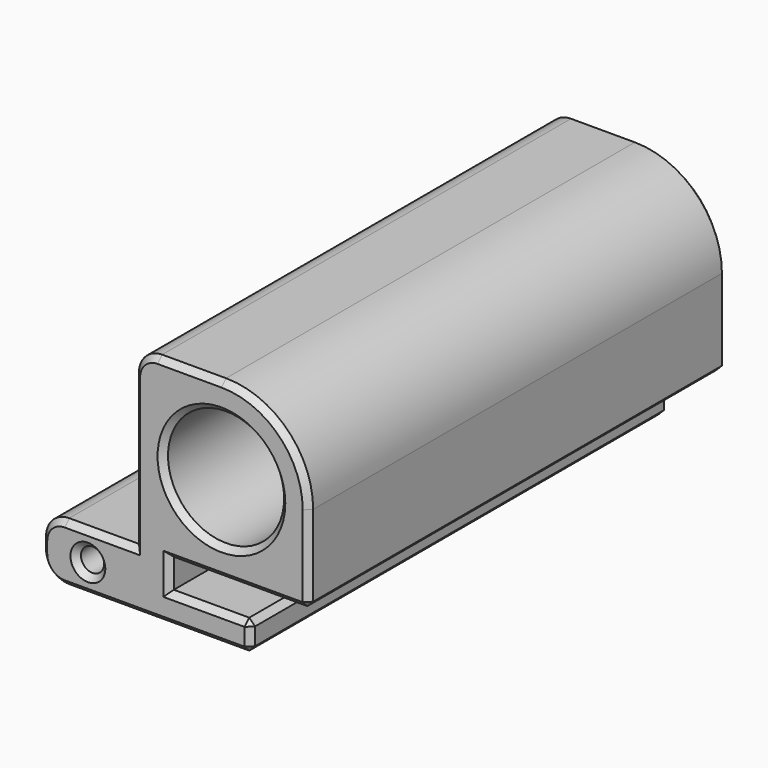
from build123d import *

# Parameters (mm, degrees)
F0_W      = 15
F0_H      = 15
F1_DEPTH  = 45
F2_R      = 5
F3_DEPTH  = 45
F4_R      = 7.5
F6_W      = 10
F6_H      = 5
F7_DEPTH  = 45
F8_W      = 7
F8_H      = 2.5
F9_DEPTH  = 45
F10_W     = 15
F10_H     = 5
F11_DEPTH = 8
F12_W     = 15
F12_H     = 5
F13_DEPTH = 8
F14_R     = 1
F15_DEPTH = 45
F16_R     = 2
F17_SIZE  = 0.5


with BuildPart() as f1:
    # F0 (on Front) → F1 (new body)
    with BuildSketch(Plane.XZ):
        with Locations((7.5, 7.5)):
            Rectangle(F0_W, F0_H)
    extrude(amount=-F1_DEPTH)

    # F2 (on face) → F3 (cut)
    with BuildSketch(Plane.XZ):
        with Locations((7.5, 7.5)):
            Circle(F2_R)
    extrude(amount=-F3_DEPTH, mode=Mode.SUBTRACT)

    # F4
    f4_edges = [f1.edges().sort_by_distance(p)[0] for p in [
        (15, 22.5, 15),
    ]]
    fillet(f4_edges, radius=F4_R)

    # F6 (on face) → F7 (join)
    with BuildSketch(Plane.XZ):
        with Locations((5, -2.5)):
            Rectangle(F6_W, F6_H)
    extrude(amount=-F7_DEPTH)

    # F8 (on face) → F9 (cut)
    with BuildSketch(Plane.XZ):
        with Locations((6.5, -1.25)):
            Rectangle(F8_W, F8_H)
    extrude(amount=-F9_DEPTH, mode=Mode.SUBTRACT)

    # F10 (on face) → F11 (join)
    with BuildSketch(Plane(origin=(0, 0, 0), x_dir=(0, -1, 0), z_dir=(-1, 0, 0))):
        with Locations((-7.5, -2.5)):
            Rectangle(F10_W, F10_H)
    extrude(amount=F11_DEPTH)

    # F12 (on face) → F13 (join)
    with BuildSketch(Plane(origin=(0, 0, 0), x_dir=(0, -1, 0), z_dir=(-1, 0, 0))):
        with Locations((-37.5, -2.5)):
            Rectangle(F12_W, F12_H)
    extrude(amount=F13_DEPTH)

    # F14 (on face) → F15 (cut)
    with BuildSketch(Plane(origin=(0, 45, 0), x_dir=(-1, 0, 0), z_dir=(0, 1, 0))):
        with Locations((4, -2.5)):
            Circle(F14_R)
    extrude(amount=-F15_DEPTH, mode=Mode.SUBTRACT)

    # F16
    f16_edges = [f1.edges().sort_by_distance(p)[0] for p in [
        (-8, 37.5, 0),
        (-8, 37.5, -5),
        (-8, 7.5, -5),
        (-8, 7.5, 0),
        (0, 22.5, 15),
    ]]
    fillet(f16_edges, radius=F16_R)

    # F17
    f17_edges = [f1.edges().sort_by_distance(p)[0] for p in [
        (0, 0, 6.5),
        (-3, 0, 0),
        (10, 0, -3.75),
        (6.5, 0, -2.5),
        (3, 0, -1.25),
        (9, 0, 0),
        (2.5, 0, 7.5),
        (-3, 15, -5),
        (-3, 15, -2.5),
        (-3, 0, -2.5),
        (-3, 30, -2.5),
        (2, 0, -5),
        (-7.414214, 45, -4.414214),
        (10, 45, -3.75),
        (6.5, 45, -2.5),
        (3, 45, -1.25),
        (9, 45, 0),
        (2.5, 45, 7.5),
        (15, 45, 3.75),
        (-3, 45, -2.5),
        (15, 22.5, 0),
        (10, 22.5, -5),
        (10, 22.5, -2.5),
        (0, 22.5, -5),
        (4.75, 0, 15),
        (4.75, 45, 15),
        (0.585786, 0, 14.414214),
        (12.803301, 0, 12.803301),
        (15, 0, 3.75),
        (-7.414214, 0, -0.585786),
        (-8, 0, -2.5),
        (-7.414214, 0, -4.414214),
        (0.585786, 45, 14.414214),
        (12.803301, 45, 12.803301),
        (0, 45, 6.5),
        (-3, 45, 0),
        (-7.414214, 45, -0.585786),
        (-8, 45, -2.5),
        (2, 45, -5),
        (-3, 15, 0),
        (-7.414214, 15, -0.585786),
        (-8, 15, -2.5),
        (-7.414214, 15, -4.414214),
        (-3, 30, -5),
        (-3, 30, 0),
        (-7.414214, 30, -0.585786),
        (-8, 30, -2.5),
        (-7.414214, 30, -4.414214),
    ]]
    chamfer(f17_edges, length=F17_SIZE)


solid = f1.part
